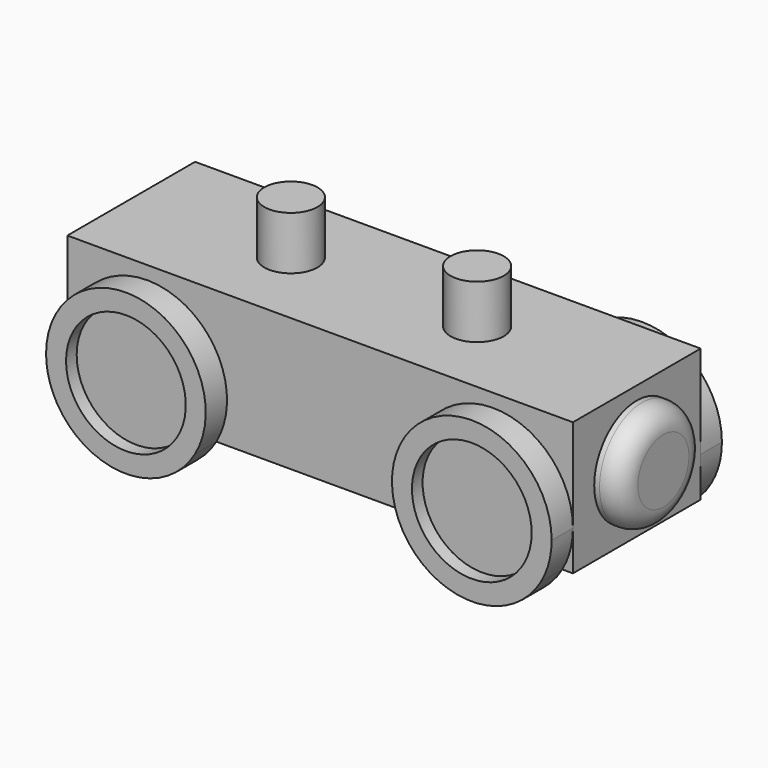
from build123d import *

# Parameters (mm, degrees)
F0_W      = 60.325
F0_H      = 15.875
F1_DEPTH  = 9.525
F3_DEPTH  = 3.175
F5_R      = 7.14375
F6_DEPTH  = 1.5875
F9_R      = 6.35
F10_DEPTH = 3.175
F11_R     = 2.54
F13_R     = 3.175
F14_DEPTH = 6.35


# Not quite as in the source:
# - a length typed as a fraction of an inch, garbled in the dataset ("3 / 203.2 mm" for 3/8 in), is restored
# - a feature names something its author has since deleted; it is built from what else it names
# - the program builds the solid bodies; features that only make, move or delete a surface that nothing else refers to are left out


with BuildPart() as f1:
    # F0 (on Front) → F1 (new body, symmetric)
    with BuildSketch(Plane.XZ):
        Rectangle(F0_W, F0_H)
    extrude(amount=F1_DEPTH, both=True)

    # F2 (on face) → F3 (join)
    with BuildSketch(Plane.XZ.offset(9.525)):
        with BuildLine():
            ThreePointArc((28.886391971, -7.9375), (29.8379434954, -5.6402514046), (30.1625, -3.175))
            ThreePointArc((30.1625, -3.175), (18.1722485954, 6.0254434954), (12.388608029, -7.9375))
            Line((12.388608029, -7.9375), (20.6375, -7.9375))
            Line((20.6375, -7.9375), (28.886391971, -7.9375))
        make_face()
        with BuildLine():
            Line((20.6375, -3.175), (20.6375, -7.9375))
            ThreePointArc((20.6375, -7.9375), (15.875, -3.175), (20.6375, 1.5875))
            Line((20.6375, 1.5875), (20.6375, -3.175))
        make_face(mode=Mode.SUBTRACT)
        with BuildLine():
            ThreePointArc((20.6375, 1.5875), (15.875, -3.175), (20.6375, -7.9375))
            Line((20.6375, -7.9375), (20.6375, -3.175))
            Line((20.6375, -3.175), (20.6375, 1.5875))
        make_face()
        with BuildLine():
            Line((20.6375, -7.9375), (12.388608029, -7.9375))
            ThreePointArc((12.388608029, -7.9375), (20.6375, -12.7), (28.886391971, -7.9375))
            Line((28.886391971, -7.9375), (20.6375, -7.9375))
        make_face()
    extrude(amount=F3_DEPTH)

    # F5 (on face) → F6 (cut)
    with BuildSketch(Plane.XZ.offset(12.7)):
        with Locations((20.6375, -3.175)):
            Circle(F5_R)
    extrude(amount=-F6_DEPTH, mode=Mode.SUBTRACT)


with BuildPart() as f7_1:
    # F7: instance of F1
    add(f1.part.mirror(Plane.YZ))


with BuildPart() as f8_1:
    # F8: instance of F1
    add(f1.part.mirror(Plane.XZ))


with BuildPart() as f8_2:
    # F8: instance of F7_1
    add(f7_1.part.mirror(Plane.XZ))


with BuildPart() as f1_1:
    add(f1.part)

    add(f7_1.part)  # F10 merges F7_1

    add(f8_1.part)  # F10 merges F8_1

    add(f8_2.part)  # F10 merges F8_2
    # F9 (on face) → F10 (join)
    with BuildSketch(Plane(origin=(-30.1625, 0, 0), x_dir=(0, -1, 0), z_dir=(-1, 0, 0))):
        Circle(F9_R)
    extrude(amount=F10_DEPTH)

    # F11
    f11_edges = [f1_1.edges().sort_by_distance(p)[0] for p in [
        (-33.3375, 6.35, 0),
    ]]
    fillet(f11_edges, radius=F11_R)


with BuildPart() as f12_1:
    # F12: instance of F1
    add(f1_1.part.mirror(Plane.YZ))


with BuildPart() as f1_2:
    add(f1_1.part)

    add(f12_1.part)  # F14 merges F12_1
    # F13 (on face) → F14 (join)
    with BuildSketch(Plane.XY.offset(7.9375)):
        with Locations((-11.1125, 0)):
            Circle(F13_R)
        with Locations((11.1125, 0)):
            Circle(F13_R)
    extrude(amount=F14_DEPTH)


solid = f1_2.part
